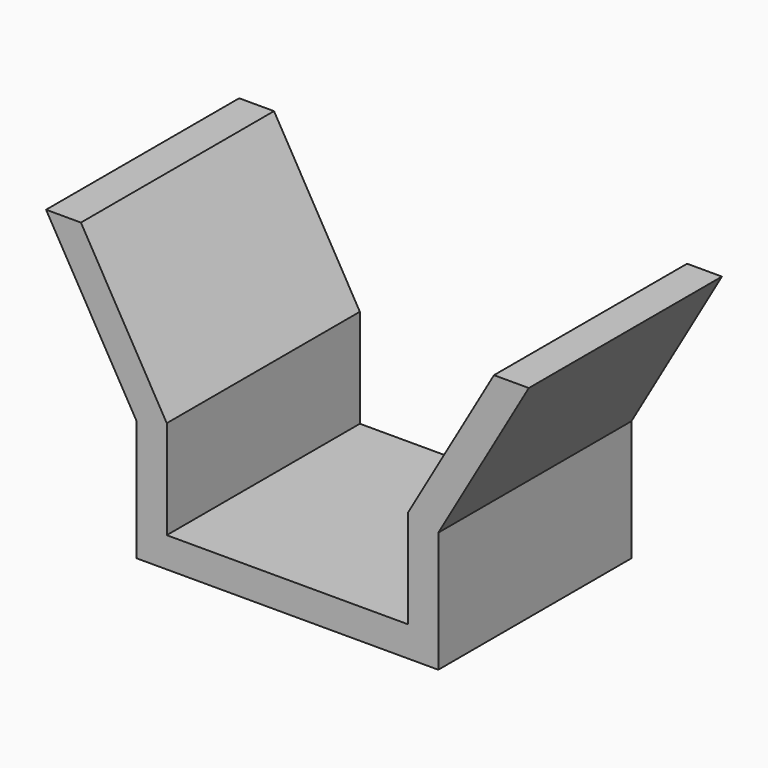
from build123d import *

# Parameters (mm, degrees)
F1_DEPTH = 50.8


# Not quite as in the source:
# - the program builds the solid bodies; features that only make, move or delete a surface that nothing else refers to are left out


with BuildPart() as f1:
    # F0 (on Front) → F1 (new body, symmetric)
    with BuildSketch(Plane.XZ):
        Polygon((-63.5, -50.8), (0, -50.8), (63.5, -50.8), (63.5, 0), (101.6, 65.9911357684), (86.9353031626, 65.9911357684), (50.8, 3.4029547439), (50.8, -38.1), (0, -38.1), (-50.8, -38.1), (-50.8, 3.4029547439), (-86.9353031626, 65.9911357684), (-101.6, 65.9911357684), (-63.5, 0), align=None)
    extrude(amount=F1_DEPTH, both=True)


solid = f1.part
